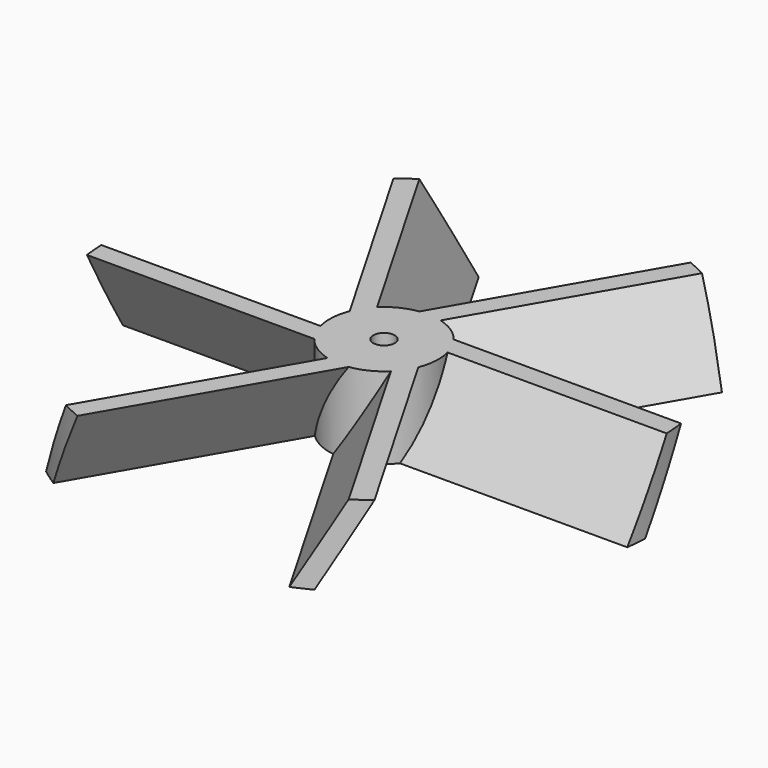
from build123d import *

# Parameters (mm, degrees)
F0_R            = 6.35
F0_R_2          = 1.24968
F1_DEPTH        = 4.7625
F4_COPIES_COUNT = 6
F5_R            = 254
F5_R_2          = 31.75
F6_DEPTH        = 9.526


# Not quite as in the source:
# - a pattern or mirror of a feature is missing from the dataset's text; its kind, count and spacing are read off the source's solid


with BuildPart() as f1:
    # F0 (on Top) → F1 (new body, symmetric)
    with BuildSketch(Plane.XY):
        Circle(F0_R)
        Circle(F0_R_2, mode=Mode.SUBTRACT)
    extrude(amount=F1_DEPTH, both=True)

    # F3 (on offset) → F4 (join, up to the next surface of F1)
    with BuildSketch(Plane.YZ.offset(152.4)):
        Polygon((1.57645491, 4.7625), (-3.922806404, -4.7625), (-1.57645491, -4.7625), (3.922806404, 4.7625), align=None)
    f4 = extrude(until=Until.NEXT, dir=(-1, 0, 0))

    # F4_copies: F4 ×6 about axis
    f4_copies_axis = Axis((0, 0, 0), (0, 0, 1))
    for i in range(1, F4_COPIES_COUNT):
        add(f4.rotate(f4_copies_axis, i * 360 / F4_COPIES_COUNT))

    # F5 (on face) → F6 (cut, through all)
    with BuildSketch(Plane.XY.offset(4.7625)):
        Circle(F5_R)
        Circle(F5_R_2, mode=Mode.SUBTRACT)
    extrude(amount=-F6_DEPTH, mode=Mode.SUBTRACT)


solid = f1.part
